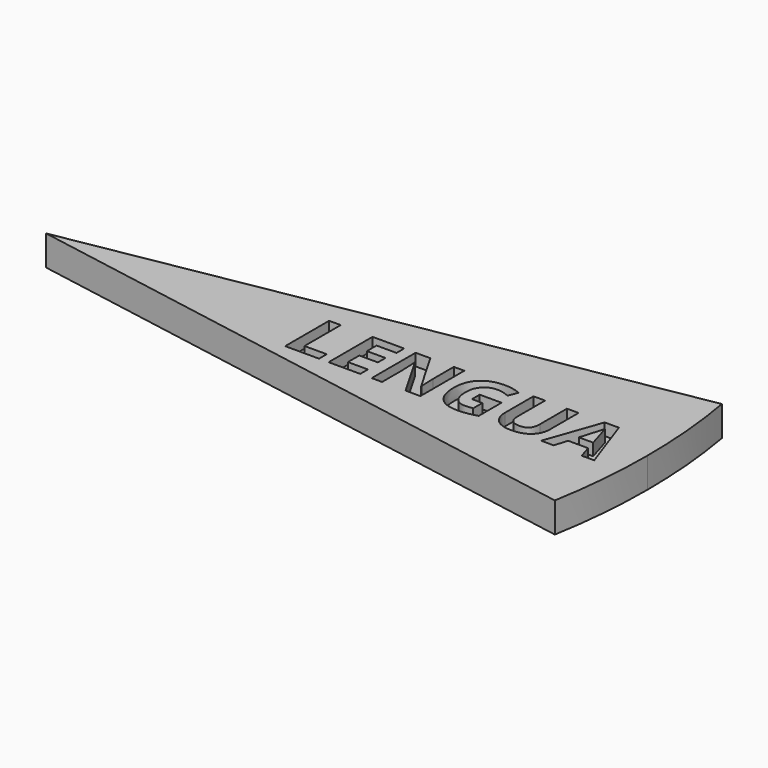
from build123d import *

# Parameters (mm, degrees)
F1_DEPTH     = 5
F2_TEXT_SIZE = 12.7900983595
F3_DEPTH     = 2


# Not quite as in the source:
# - Text() gives the source's letters only with a copy of the font that has no kerning and outlines rounded to 1/6400 em; it was checked with that copy


with BuildPart() as f1:
    # F0 (on Top) → F1 (new body)
    with BuildSketch(Plane.XY):
        with BuildLine():
            Line((0, 0), (98.4807753012, -17.3648177667))
            ThreePointArc((98.4807753012, -17.3648177667), (99.6194698092, -8.7155742748), (100, 0))
            Line((100, 0), (0, 0))
        make_face()
        with BuildLine():
            Line((0, 0), (100, 0))
            ThreePointArc((100, 0), (99.6194698092, 8.7155742748), (98.4807753012, 17.3648177667))
            Line((98.4807753012, 17.3648177667), (0, 0))
        make_face()
    extrude(amount=F1_DEPTH)

    # F2 (on face) → F3 (cut)
    with BuildSketch(Plane.XY.offset(5)):
        with Locations((42.8876131773, -5.3610184696)):
            Text('LENGUA', F2_TEXT_SIZE, font='Open Sans', font_style=FontStyle.BOLD, text_align=(TextAlign.LEFT, TextAlign.BOTTOM))
    extrude(amount=-F3_DEPTH, mode=Mode.SUBTRACT)


solid = f1.part
